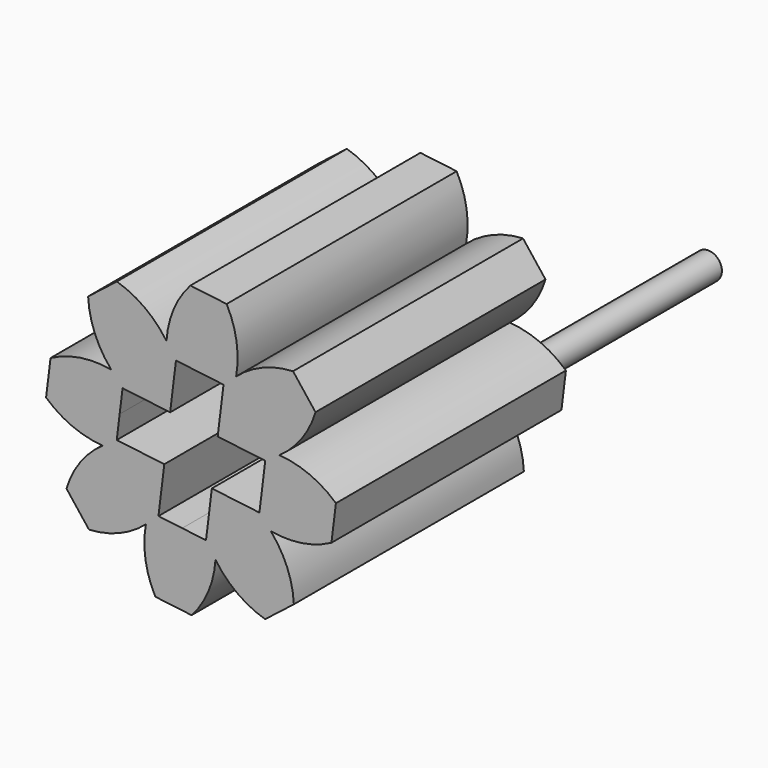
from build123d import *

# Parameters (mm, degrees)
F2_R            = 1.46
F3_DEPTH        = 8
F4_DEPTH        = 8
F4_COPIES_COUNT = 8
F6_DEPTH        = 25.4
F7_R            = 0.3801945308
F8_DEPTH        = 6.35


# Not quite as in the source:
# - a pattern or mirror of a feature is missing from the dataset's text; its kind, count and spacing are read off the source's solid


with BuildPart() as f3:
    # F2 (on Front) → F3 (new body)
    with BuildSketch(Plane.XZ):
        Circle(F2_R)
    extrude(amount=F3_DEPTH)

    # F0 (on Front) → F4 (join, through all)
    with BuildSketch(Plane.XZ):
        with BuildLine():
            Line((0.9916843511, 3.9082757742), (-0.016742539, 4.0320950271))
            ThreePointArc((-0.016742539, 4.0320950271), (-0.4815870331, 3.3038967388), (-0.6807987002, 2.4632613466))
            Line((-0.6807987002, 2.4632613466), (-0.7599388939, 1.2466326153))
            ThreePointArc((-0.7599388939, 1.2466326153), (0.1779282969, 1.4491174974), (1.0389518493, 1.0257577954))
            Line((1.0389518493, 1.0257577954), (1.2564873073, 2.2253939754))
            ThreePointArc((1.2564873073, 2.2253939754), (1.2665577946, 3.089252966), (0.9916843511, 3.9082757742))
        make_face()
    f4 = extrude(amount=F4_DEPTH)

    # F4_copies: F4 ×8 about axis
    f4_copies_axis = Axis((0, 0, 0), (0, 1, 0))
    for i in range(1, F4_COPIES_COUNT):
        add(f4.rotate(f4_copies_axis, i * 360 / F4_COPIES_COUNT))

    # F5 (on Front) → F6 (cut)
    with BuildSketch(Plane.XZ):
        Polygon((0.7429379899, 0.5804584672), (0.9054304478, 1.9038533361), (0.2437330133, 1.985099565), (-0.4179644211, 2.0663457939), (-0.580456879, 0.7429509251), (-1.9038517478, 0.9054433829), (-1.9850979768, 0.2437459485), (-2.0663442057, -0.4179514859), (-0.7429493368, -0.5804439438), (-0.9054417947, -1.9038388126), (-0.2437443603, -1.9850850416), (0.4179530741, -2.0663312705), (0.580445532, -0.7429364017), (1.9038404009, -0.9054288595), (1.9850866298, -0.2437314251), (2.0663328587, 0.4179660093), align=None)
    extrude(amount=F6_DEPTH, mode=Mode.SUBTRACT)

    # F7 (on Front) → F8 (join)
    with BuildSketch(Plane.XZ):
        with Locations((2.9130612966, -0.3662490635)):
            Circle(F7_R)
    extrude(amount=-F8_DEPTH)


solid = f3.part
